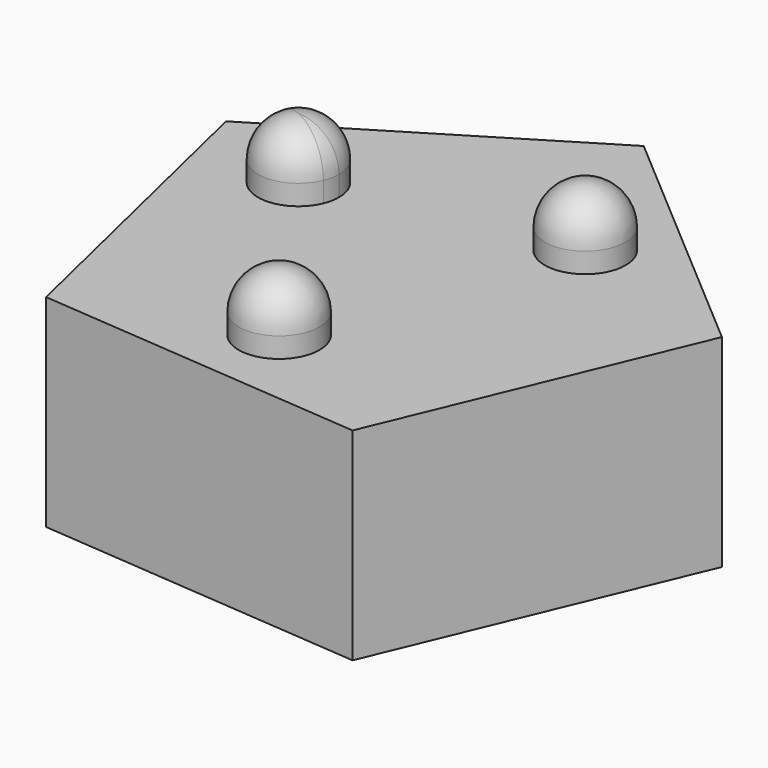
from build123d import *

# Parameters (mm, degrees)
F0_R     = 10
F1_DEPTH = 50
F2_DEPTH = 65
F3_R     = 10


with BuildPart() as f1:
    # F0 (on Top) → F1 (new body)
    with BuildSketch(Plane.XY):
        Polygon((35.9642069631, -59.0012792924), (67.2271022816, 15.9715953944), (5.5844272121, 68.8722681007), (-63.7757364568, 26.5938071741), (-45, -52.4363913769), align=None)
        with Locations((0, -36.73)):
            Circle(F0_R, mode=Mode.SUBTRACT)
        with BuildLine():
            ThreePointArc((-27.689133859, 11.5460757896), (-40.7675370752, 6.1650564331), (-46.1485564317, 19.2434596493))
            ThreePointArc((-46.1485564317, 19.2434596493), (-34.9563356375, 25.2003047486), (-26.9188451453, 15.3947677194))
            ThreePointArc((-26.9188451453, 15.3947677194), (-27.1133081161, 13.4322582116), (-27.689133859, 11.5460757896))
        make_face(mode=Mode.SUBTRACT)
        with Locations((23.9935845951, 27.8100844709)):
            Circle(F0_R, mode=Mode.SUBTRACT)
    extrude(amount=F1_DEPTH)

    # F0 (on Top) → F2 (join)
    with BuildSketch(Plane.XY):
        with BuildLine():
            Line((-27.689133859, 11.5460757896), (-46.1485564317, 19.2434596493))
            ThreePointArc((-46.1485564317, 19.2434596493), (-40.7675370752, 6.1650564331), (-27.689133859, 11.5460757896))
        make_face()
        with BuildLine():
            ThreePointArc((-26.9188451453, 15.3947677194), (-34.9563356375, 25.2003047486), (-46.1485564317, 19.2434596493))
            Line((-46.1485564317, 19.2434596493), (-27.689133859, 11.5460757896))
            ThreePointArc((-27.689133859, 11.5460757896), (-27.1133081161, 13.4322582116), (-26.9188451453, 15.3947677194))
        make_face()
        with Locations((23.9935845951, 27.8100844709)):
            Circle(F0_R)
        with Locations((0, -36.73)):
            Circle(F0_R)
    extrude(amount=F2_DEPTH)

    # F3
    f3_edges = [f1.edges().sort_by_distance(p)[0] for p in [
        (-46.148556, 19.24346, 65),
        (-10, -36.73, 65),
        (13.993585, 27.810084, 65),
    ]]
    fillet(f3_edges, radius=F3_R)


solid = f1.part
